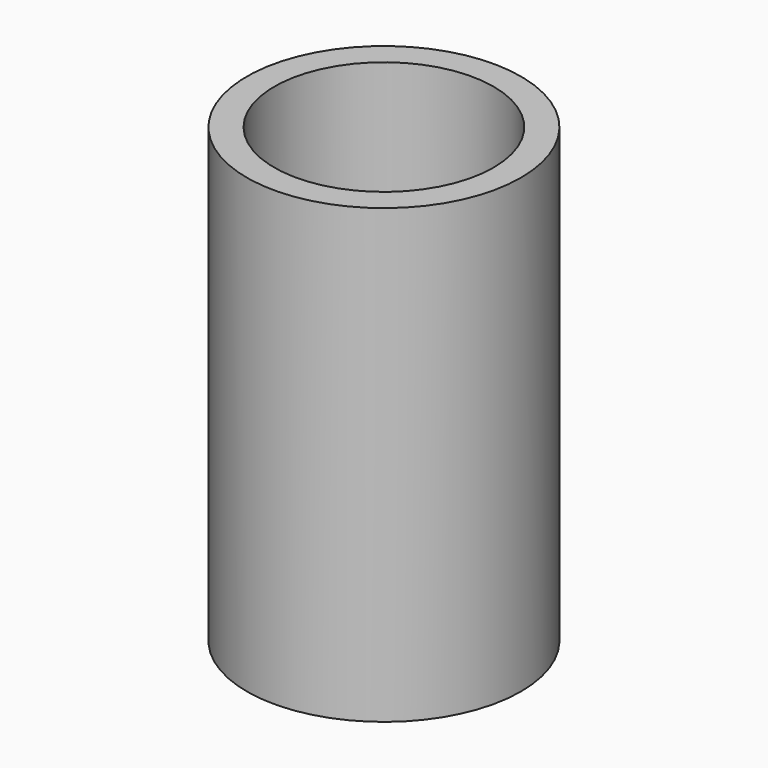
from build123d import *

# Parameters (mm, degrees)
F0_R     = 5
F0_R_2   = 4
F1_DEPTH = 15
F2_R     = 5
F3_DEPTH = 1.5
F4_W     = 1.2
F4_H     = 6.4
F5_DEPTH = 2
F6_W     = 0.8
F6_H     = 4
F7_DEPTH = 2


# Not quite as in the source:
# - a pattern or mirror of a feature is missing from the dataset's text; its kind, count and spacing are read off the source's solid


with BuildPart() as f1:
    # F0 (on Top) → F1 (new body)
    with BuildSketch(Plane.XY):
        Circle(F0_R)
        Circle(F0_R_2, mode=Mode.SUBTRACT)
    extrude(amount=F1_DEPTH)

    # F2 (on Top) → F3 (join)
    with BuildSketch(Plane.XY):
        Circle(F2_R)
    extrude(amount=-F3_DEPTH)

    # F4 (on Top) → F5 (cut)
    with BuildSketch(Plane.XY):
        Rectangle(F4_W, F4_H)
    extrude(amount=-F5_DEPTH, mode=Mode.SUBTRACT)

    # F6 (on Top) → F7 (join)
    with BuildSketch(Plane.XY):
        with Locations((2.4, 0)):
            Rectangle(F6_W, F6_H)
    f7 = extrude(amount=F7_DEPTH)

    # F7_copies: F7 across plane
    add(f7.mirror(Plane(origin=(0, 0, 0), x_dir=(0, 0, -1), z_dir=(-1, 0, 0))))


solid = f1.part
